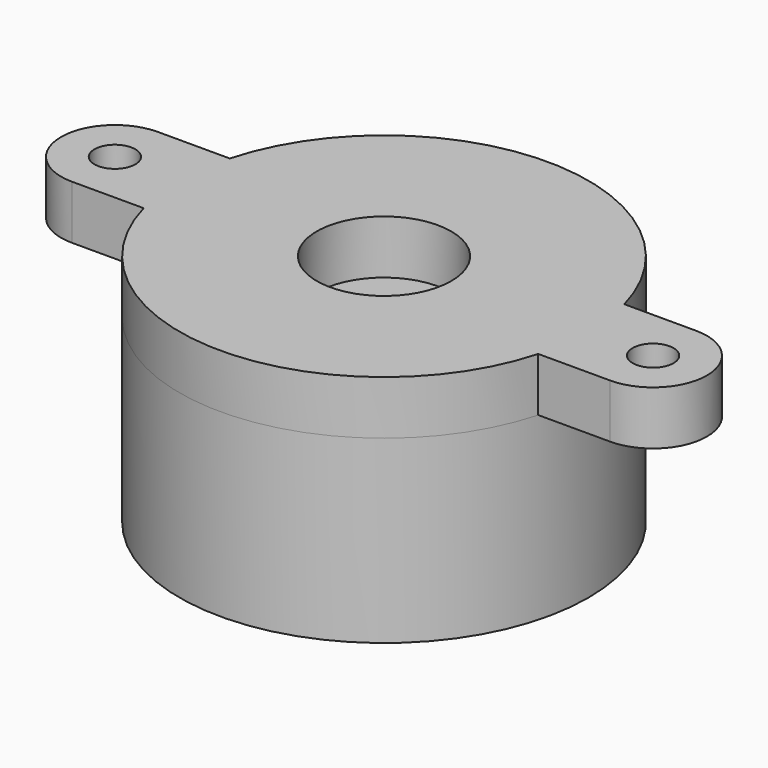
from build123d import *

# Parameters (mm, degrees)
F0_R     = 24.13
F0_R_2   = 20.955
F1_DEPTH = 16.51
F2_R     = 18.415
F2_R_2   = 24.13
F4_DEPTH = 4.7625
F5_R     = 3.96875
F6_DEPTH = 4.7625
F5_R_2   = 2.413
F5_R_3   = 7.9375
F7_DEPTH = 6.35


# Not quite as in the source:
# - a feature names something its author has since deleted; it is built from what else it names


with BuildPart() as f1:
    # F0 (on Top) → F1 (new body)
    with BuildSketch(Plane.XY):
        Circle(F0_R)
        Circle(F0_R_2, mode=Mode.SUBTRACT)
        Circle(F0_R_2)
    extrude(amount=F1_DEPTH)

    # F0 (on Top) → F3 section 0
    with BuildSketch(Plane.XY):
        Circle(F0_R_2)
    # F2 (on face) → F3 section 1
    with BuildSketch(Plane.XY.offset(16.51)):
        Circle(F2_R)
    loft(mode=Mode.SUBTRACT)

    # F2 (on face) → F4 (join)
    with BuildSketch(Plane.XY.offset(16.51)):
        Circle(F2_R_2)
        Circle(F2_R, mode=Mode.SUBTRACT)
        Circle(F2_R)
    extrude(amount=F4_DEPTH)

    # F5 (on face) → F6 (cut, through all)
    with BuildSketch(Plane.XY.offset(21.2725)):
        Circle(F5_R)
    extrude(amount=-F6_DEPTH, mode=Mode.SUBTRACT)

    # F5 (on face) → F7 (join)
    with BuildSketch(Plane.XY.offset(21.2725)):
        with BuildLine():
            Line((-26.2298047315, 6.35), (-31.75, 6.35))
            ThreePointArc((-31.75, 6.35), (-38.1, 0), (-31.75, -6.35))
            Line((-31.75, -6.35), (-26.2298047315, -6.35))
            ThreePointArc((-26.2298047315, -6.35), (-26.9875, 0), (-26.2298047315, 6.35))
        make_face()
        with Locations((-31.75, 0)):
            Circle(F5_R_2, mode=Mode.SUBTRACT)
        with BuildLine():
            ThreePointArc((23.2794845304, 6.35), (0, 24.13), (-23.2794845304, 6.35))
            ThreePointArc((-23.2794845304, 6.35), (-24.13, 0), (-23.2794845304, -6.35))
            ThreePointArc((-23.2794845304, -6.35), (0, -24.13), (23.2794845304, -6.35))
            ThreePointArc((23.2794845304, -6.35), (23.9164259633, -3.2033527968), (24.13, 0))
            ThreePointArc((24.13, 0), (23.9164259633, 3.2033527968), (23.2794845304, 6.35))
        make_face()
        Circle(F5_R_3, mode=Mode.SUBTRACT)
        with BuildLine():
            Line((31.75, 6.35), (26.2298047315, 6.35))
            ThreePointArc((26.2298047315, 6.35), (26.9875, 0), (26.2298047315, -6.35))
            Line((26.2298047315, -6.35), (31.75, -6.35))
            ThreePointArc((31.75, -6.35), (38.1, 0), (31.75, 6.35))
        make_face()
        with Locations((31.75, 0)):
            Circle(F5_R_2, mode=Mode.SUBTRACT)
        with BuildLine():
            Line((-23.2794845304, 6.35), (-26.2298047315, 6.35))
            ThreePointArc((-26.2298047315, 6.35), (-26.9875, 0), (-26.2298047315, -6.35))
            Line((-26.2298047315, -6.35), (-23.2794845304, -6.35))
            ThreePointArc((-23.2794845304, -6.35), (-24.13, 0), (-23.2794845304, 6.35))
        make_face()
        with BuildLine():
            Line((26.2298047315, 6.35), (23.2794845304, 6.35))
            ThreePointArc((23.2794845304, 6.35), (23.9164259633, 3.2033527968), (24.13, 0))
            ThreePointArc((24.13, 0), (23.9164259633, -3.2033527968), (23.2794845304, -6.35))
            Line((23.2794845304, -6.35), (26.2298047315, -6.35))
            ThreePointArc((26.2298047315, -6.35), (26.9875, 0), (26.2298047315, 6.35))
        make_face()
    extrude(amount=F7_DEPTH)


solid = f1.part
